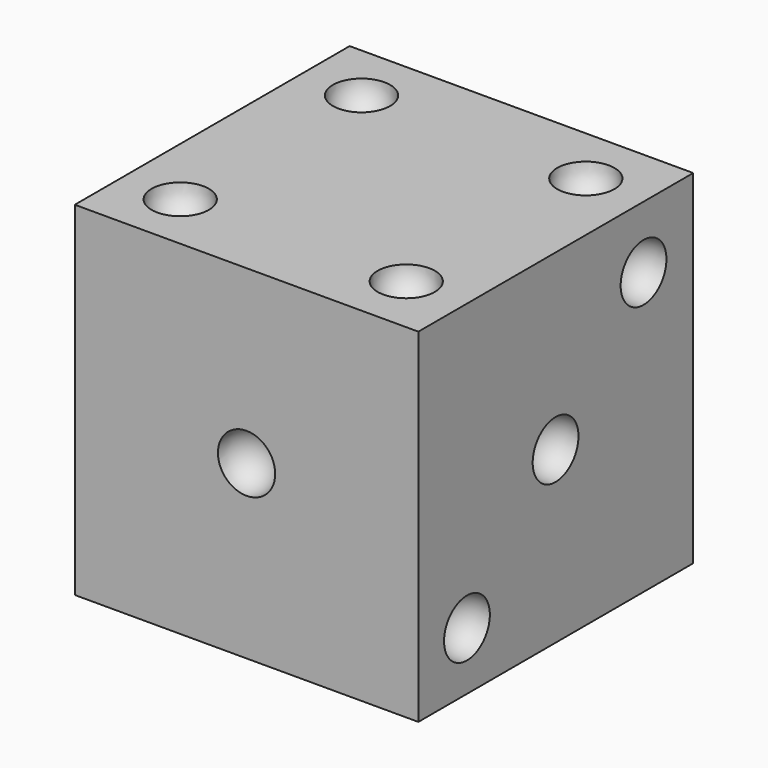
from build123d import *

# Parameters (mm, degrees)
F0_W     = 76.2
F0_H     = 76.2
F1_DEPTH = 76.2


# Not quite as in the source:
# - a feature names something its author has since deleted; it is built from what else it names


with BuildPart() as f1:
    # F0 (on Front) → F1 (new body)
    with BuildSketch(Plane.XZ):
        with Locations((-38.1, 38.1)):
            Rectangle(F0_W, F0_H)
    extrude(amount=F1_DEPTH)

    # F2 (on face) → F3 (revolve, cut)
    with BuildSketch(Plane.XZ.offset(76.2)):
        with BuildLine():
            Line((-38.1, 44.45), (-38.1, 31.75))
            ThreePointArc((-38.1, 31.75), (-31.75, 38.1), (-38.1, 44.45))
        make_face()
    revolve(axis=Axis((-38.1, -76.2, 38.1), (0, 0, -1)), mode=Mode.SUBTRACT)

    # F4 (on Right) → F6 (revolve, cut)
    with BuildSketch(Plane.YZ):
        with BuildLine():
            ThreePointArc((-42.6203764111, 33.2101642958), (-33.6402650036, 33.261145749), (-33.6912464568, 42.2412571565))
            Line((-33.6912464568, 42.2412571565), (-42.6203764111, 33.2101642958))
        make_face()
        with BuildLine():
            ThreePointArc((-18.2330377902, 57.8759851359), (-9.2529263827, 57.9269665892), (-9.303907836, 66.9070779967))
            Line((-9.303907836, 66.9070779967), (-18.2330377902, 57.8759851359))
        make_face()
        with BuildLine():
            ThreePointArc((-67.1930310408, 8.356911299), (-58.2129196333, 8.4078927522), (-58.2639010865, 17.3880041597))
            Line((-58.2639010865, 17.3880041597), (-67.1930310408, 8.356911299))
        make_face()
    revolve(axis=Axis((0, -37.7277955413, 38.1586141884), (0, -0.7030810988, -0.7111096741)), mode=Mode.SUBTRACT)

    # F5 (on face) → F7 (revolve, cut)
    with BuildSketch(Plane(origin=(0, 0, 0), x_dir=(-1, 0, 0), z_dir=(0, 1, 0))):
        with BuildLine():
            ThreePointArc((13.3039106504, 62.8960893496), (13.3039106504, 71.8763454707), (4.3236545293, 71.8763454707))
            Line((4.3236545293, 71.8763454707), (13.3039106504, 62.8960893496))
        make_face()
        with BuildLine():
            Line((62.2215412564, 13.9784587436), (71.2017973774, 4.9982026226))
            ThreePointArc((71.2017973774, 4.9982026226), (71.2017973774, 13.9784587436), (62.2215412564, 13.9784587436))
        make_face()
    revolve(axis=Axis((-38.1, 0, 38.1), (-0.7071067812, 0, -0.7071067812)), mode=Mode.SUBTRACT)

    # F8 (on face) → F9 (revolve, cut)
    with BuildSketch(Plane(origin=(0, 0, 0), x_dir=(1, 0, 0), z_dir=(0, 0, -1))):
        with BuildLine():
            Line((-7.6989389031, 68.5010610969), (-16.6791950242, 59.5208049758))
            ThreePointArc((-16.6791950242, 59.5208049758), (-9.7590271681, 58.1442980049), (-5.8390669636, 64.0109330364))
            ThreePointArc((-5.8390669636, 64.0109330364), (-6.3224319322, 66.4409728319), (-7.6989389031, 68.5010610969))
        make_face()
        with BuildLine():
            ThreePointArc((-55.5683625042, 14.2816374958), (-56.0517274728, 16.7116772913), (-57.4282344437, 18.7717655563))
            Line((-57.4282344437, 18.7717655563), (-66.4084905648, 9.7915094352))
            ThreePointArc((-66.4084905648, 9.7915094352), (-59.4883227087, 8.4150024643), (-55.5683625042, 14.2816374958))
        make_face()
    revolve(axis=Axis((-38.1, -38.1, 0), (0.7071067812, -0.7071067812, 0)), mode=Mode.SUBTRACT)

    # F11 (on face) → F12 (revolve, cut)
    with BuildSketch(Plane(origin=(0, 0, 0), x_dir=(-1, 0, 0), z_dir=(0, 1, 0))):
        with BuildLine():
            ThreePointArc((33.6098719395, 33.6098719395), (42.5901280605, 33.6098719395), (42.5901280605, 42.5901280605))
            Line((42.5901280605, 42.5901280605), (33.6098719395, 33.6098719395))
        make_face()
        with BuildLine():
            Line((17.1070893237, 17.1070893237), (8.1268332026, 8.1268332026))
            ThreePointArc((8.1268332026, 8.1268332026), (17.1070893237, 8.1268332026), (17.1070893237, 17.1070893237))
        make_face()
        with BuildLine():
            ThreePointArc((61.5488939977, 61.5488939977), (70.5291501188, 61.5488939977), (70.5291501188, 70.5291501188))
            Line((70.5291501188, 70.5291501188), (61.5488939977, 61.5488939977))
        make_face()
    revolve(axis=Axis((-38.1, 0, 38.1), (0.7071067812, 0, -0.7071067812)), mode=Mode.SUBTRACT)

    # F10 (on face) → F13 (revolve, cut)
    with BuildSketch(Plane.XY.offset(76.2)):
        with BuildLine():
            Line((-17.9101203458, -58.2898796542), (-8.9298642247, -67.2701357753))
            ThreePointArc((-8.9298642247, -67.2701357753), (-8.9298642247, -58.2898796542), (-17.9101203458, -58.2898796542))
        make_face()
        with BuildLine():
            Line((-67.516321119, -8.683678881), (-58.536064998, -17.663935002))
            ThreePointArc((-58.536064998, -17.663935002), (-58.536064998, -8.683678881), (-67.516321119, -8.683678881))
        make_face()
    revolve(axis=Axis((-38.1, -38.1, 76.2), (-0.7071067812, 0.7071067812, 0)), mode=Mode.SUBTRACT)

    # F14 (on face) → F15 (revolve, cut)
    with BuildSketch(Plane.XY.offset(76.2)):
        with BuildLine():
            Line((-67.6980300748, -67.6980300748), (-58.7177739537, -58.7177739537))
            ThreePointArc((-58.7177739537, -58.7177739537), (-67.6980300748, -58.7177739537), (-67.6980300748, -67.6980300748))
        make_face()
        with BuildLine():
            Line((-17.7225505875, -17.7225505875), (-8.7422944664, -8.7422944664))
            ThreePointArc((-8.7422944664, -8.7422944664), (-17.7225505875, -8.7422944664), (-17.7225505875, -17.7225505875))
        make_face()
    revolve(axis=Axis((-38.1, -38.1, 76.2), (-0.7071067812, -0.7071067812, 0)), mode=Mode.SUBTRACT)

    # F16 (on face) → F17 (revolve, cut)
    with BuildSketch(Plane(origin=(-76.2, 0, 0), x_dir=(0, -1, 0), z_dir=(-1, 0, 0))):
        with BuildLine():
            ThreePointArc((18.8331212848, 57.9041870475), (25.1831212848, 64.2541870475), (18.8331212848, 70.6041870475))
            Line((18.8331212848, 70.6041870475), (18.8331212848, 57.9041870475))
        make_face()
        with BuildLine():
            ThreePointArc((18.8331212848, 31.75), (25.1831212848, 38.1), (18.8331212848, 44.45))
            Line((18.8331212848, 44.45), (18.8331212848, 31.75))
        make_face()
        with BuildLine():
            Line((18.8331212848, 20.6239342076), (18.8331212848, 7.933481844))
            ThreePointArc((18.8331212848, 7.933481844), (24.9369410634, 14.2787080258), (18.8331212848, 20.6239342076))
        make_face()
    revolve(axis=Axis((-76.2, -18.8331212848, 38.1), (0, 0, -1)), mode=Mode.SUBTRACT)

    # F18 (on face) → F19 (revolve, cut)
    with BuildSketch(Plane(origin=(-76.2, 0, 0), x_dir=(0, -1, 0), z_dir=(-1, 0, 0))):
        with BuildLine():
            ThreePointArc((56.007001549, 59.3812944531), (62.357001549, 65.7312944531), (56.007001549, 72.0812944531))
            Line((56.007001549, 72.0812944531), (56.007001549, 59.3812944531))
        make_face()
        with BuildLine():
            ThreePointArc((56.007001549, 31.75), (62.357001549, 38.1), (56.007001549, 44.45))
            Line((56.007001549, 44.45), (56.007001549, 31.75))
        make_face()
        with BuildLine():
            Line((56.007001549, 20.6287080258), (56.007001549, 7.9287080258))
            ThreePointArc((56.007001549, 7.9287080258), (62.357001549, 14.2787080258), (56.007001549, 20.6287080258))
        make_face()
    revolve(axis=Axis((-76.2, -56.007001549, 38.1), (0, 0, -1)), mode=Mode.SUBTRACT)


solid = f1.part
